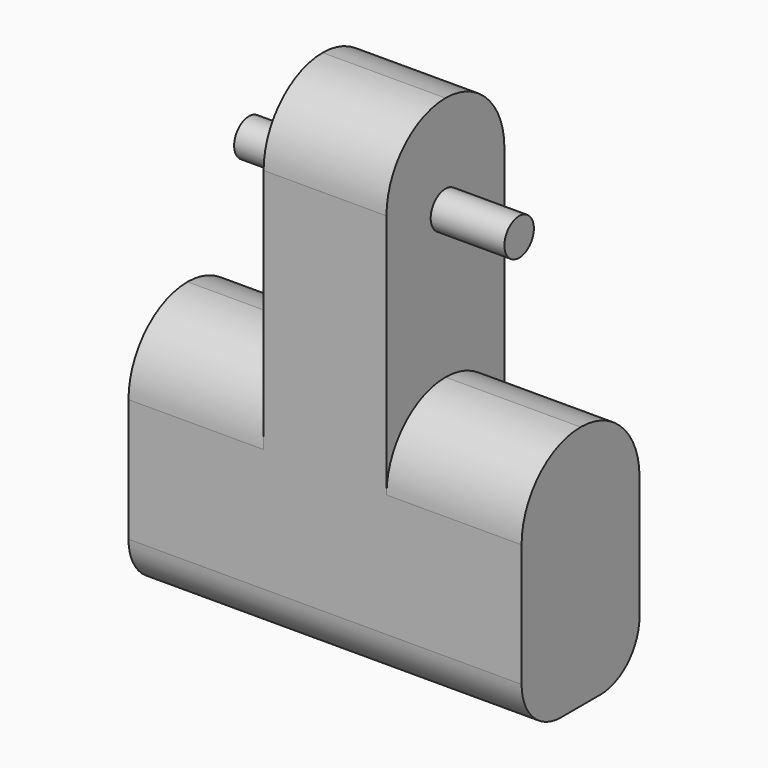
from build123d import *

# Parameters (mm, degrees)
F1_DEPTH      = 6
F2_R          = 0.75
F3_DEPTH      = 3
F3_DEPTH_BACK = 8
F4_R          = 2.99999
F5_R          = 2.99999
F6_R          = 2


# Not quite as in the source:
# - a fillet or chamfer is up to 0.001 mm smaller than in the source, because OpenCascade refuses the exact size


with BuildPart() as f1:
    # F0 (on Front) → F1 (new body)
    with BuildSketch(Plane.XZ):
        Polygon((5.5, 0), (0, 0), (0, -10), (16, -10), (16, 0), (10.5, 0), (10.5, 10), (5.5, 10), align=None)
    extrude(amount=F1_DEPTH)

    # F2 (on face) → F3 (join, two sides)
    with BuildSketch(Plane.YZ.offset(10.5)) as f3_sk:
        with Locations((-3, 6)):
            Circle(F2_R)
    extrude(amount=F3_DEPTH)
    extrude(f3_sk.sketch, amount=-F3_DEPTH_BACK)

    # F4 (radius 3 in the source; OpenCascade refuses exactly that, so slightly less here)
    f4_edges = [f1.edges().sort_by_distance(p)[0] for p in [
        (8, -6, 10),
        (8, 0, 10),
    ]]
    fillet(f4_edges, radius=F4_R)

    # F5 (radius 3 in the source; OpenCascade refuses exactly that, so slightly less here)
    f5_edges = [f1.edges().sort_by_distance(p)[0] for p in [
        (2.75, -6, 0),
        (2.75, 0, 0),
        (13.25, -6, 0),
        (13.25, 0, 0),
    ]]
    fillet(f5_edges, radius=F5_R)

    # F6
    f6_edges = [f1.edges().sort_by_distance(p)[0] for p in [
        (8, -6, -10),
        (8, 0, -10),
    ]]
    fillet(f6_edges, radius=F6_R)


solid = f1.part
